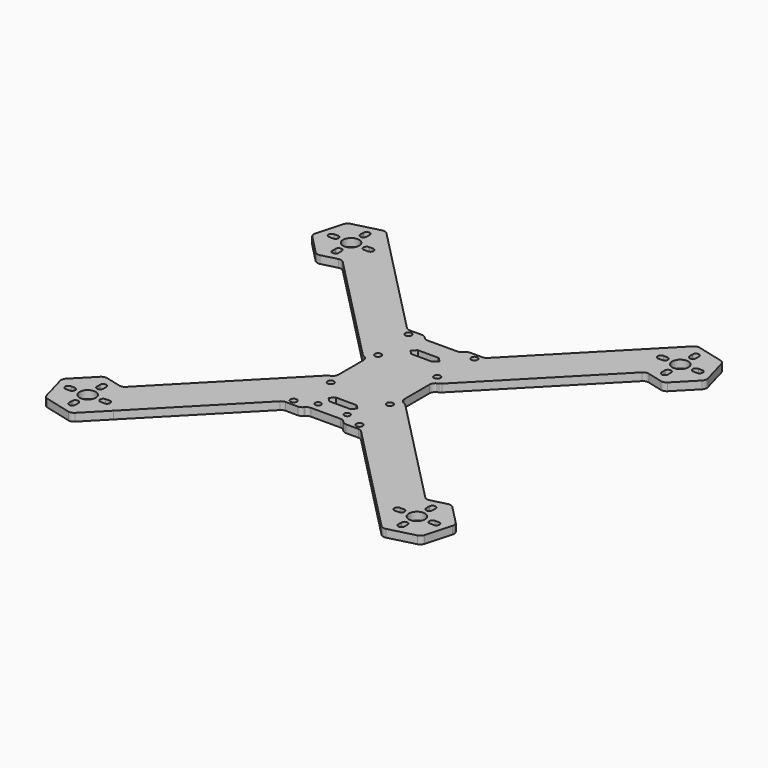
from build123d import *

# Parameters (mm, degrees)
F0_R     = 1.65
F0_R_2   = 4.15
F1_DEPTH = 4
F2_R     = 3
F5_R     = 1.5
F6_DEPTH = 43.5


# Not quite as in the source:
# - a feature names something its author has since deleted; it is built from what else it names


with BuildPart() as f1:
    # F0 (on Top) → F1 (new body)
    with BuildSketch(Plane.XY):
        Polygon((20, 40), (14, 40), (11.0626053065, 40), (9, 37.6), (0, 37.6), (0, 28.5310465842), (5.3786796564, 28.5310465842), (7.5, 26.4097262407), (5.3786796564, 24.2884058971), (0, 24.2884058971), (0, 0), (17, 0), (17, 10), (20, 11.3973480558), (78.334668641, 71.0380709735), (72.7416933404, 72.4705375943), (68.0738878405, 89.1502136048), align=None)
        with Locations((15.25, 15.25)):
            Circle(F0_R, mode=Mode.SUBTRACT)
        with Locations((17, 37)):
            Circle(F0_R, mode=Mode.SUBTRACT)
        Polygon((80.1850082425, 101.5324897529), (68.0738878405, 89.1502136048), (72.7416933404, 72.4705375943), (78.334668641, 71.0380709735), (89.5206192423, 68.1731377319), (101.6317396443, 80.55541388), (96.9639341444, 97.2350898905), align=None)
        with BuildLine():
            ThreePointArc((83.2528137424, 76.8528137424), (84.8528137424, 78.4528137424), (86.4528137424, 76.8528137424))
            Line((86.4528137424, 76.8528137424), (86.4528137424, 76.2028137424))
            Line((86.4528137424, 76.2028137424), (86.4528137424, 75.3528137424))
            Line((86.4528137424, 75.3528137424), (86.4528137424, 74.8528137424))
            ThreePointArc((86.4528137424, 74.8528137424), (84.8528137424, 73.2528137424), (83.2528137424, 74.8528137424))
            Line((83.2528137424, 74.8528137424), (83.2528137424, 76.2028137424))
            Line((83.2528137424, 76.2028137424), (83.2528137424, 76.8528137424))
        make_face(mode=Mode.SUBTRACT)
        with BuildLine():
            ThreePointArc((76.8528137424, 86.4528137424), (78.4528137424, 84.8528137424), (76.8528137424, 83.2528137424))
            Line((76.8528137424, 83.2528137424), (76.2028137424, 83.2528137424))
            Line((76.2028137424, 83.2528137424), (75.3528137424, 83.2528137424))
            Line((75.3528137424, 83.2528137424), (74.8528137424, 83.2528137424))
            ThreePointArc((74.8528137424, 83.2528137424), (73.2528137424, 84.8528137424), (74.8528137424, 86.4528137424))
            Line((74.8528137424, 86.4528137424), (76.2028137424, 86.4528137424))
            Line((76.2028137424, 86.4528137424), (76.8528137424, 86.4528137424))
        make_face(mode=Mode.SUBTRACT)
        with Locations((84.8528137424, 84.8528137424)):
            Circle(F0_R_2, mode=Mode.SUBTRACT)
        with BuildLine():
            Line((93.5028137424, 83.2528137424), (92.8528137424, 83.2528137424))
            ThreePointArc((92.8528137424, 83.2528137424), (91.2528137424, 84.8528137424), (92.8528137424, 86.4528137424))
            Line((92.8528137424, 86.4528137424), (93.5028137424, 86.4528137424))
            Line((93.5028137424, 86.4528137424), (94.8528137424, 86.4528137424))
            ThreePointArc((94.8528137424, 86.4528137424), (96.4528137424, 84.8528137424), (94.8528137424, 83.2528137424))
            Line((94.8528137424, 83.2528137424), (94.3528137424, 83.2528137424))
            Line((94.3528137424, 83.2528137424), (93.5028137424, 83.2528137424))
        make_face(mode=Mode.SUBTRACT)
        with BuildLine():
            ThreePointArc((86.4528137424, 92.8528137424), (84.8528137424, 91.2528137424), (83.2528137424, 92.8528137424))
            Line((83.2528137424, 92.8528137424), (83.2528137424, 93.5028137424))
            Line((83.2528137424, 93.5028137424), (83.2528137424, 94.3528137424))
            Line((83.2528137424, 94.3528137424), (83.2528137424, 94.8528137424))
            ThreePointArc((83.2528137424, 94.8528137424), (84.8528137424, 96.4528137424), (86.4528137424, 94.8528137424))
            Line((86.4528137424, 94.8528137424), (86.4528137424, 94.3528137424))
            Line((86.4528137424, 94.3528137424), (86.4528137424, 93.5028137424))
            Line((86.4528137424, 93.5028137424), (86.4528137424, 92.8528137424))
        make_face(mode=Mode.SUBTRACT)
    extrude(amount=F1_DEPTH)

    # F2
    f2_edges = [f1.edges().sort_by_distance(p)[0] for p in [
        (20, 11.397348, 2),
        (78.334669, 71.038071, 2),
        (17, 10, 2),
        (89.520619, 68.173138, 2),
        (101.63174, 80.555414, 2),
        (96.963934, 97.23509, 2),
        (80.185008, 101.53249, 2),
        (20, 40, 2),
        (11.062605, 40, 2),
        (9, 37.6, 2),
    ]]
    fillet(f2_edges, radius=F2_R)

    # F3: F1 across plane


with BuildPart() as f1_1:
    add(f1.part)
    add(f1.part.mirror(Plane.YZ))

    # F4: F1 across plane


with BuildPart() as f1_2:
    add(f1_1.part)
    add(f1_1.part.mirror(Plane.XZ))

    # F5 (on face) → F6 (cut, symmetric)
    with BuildSketch(Plane.XY.offset(4)):
        with Locations((-7.5, -33.0655232921)):
            Circle(F5_R)
        with Locations((7.5, -33.0655232921)):
            Circle(F5_R)
    extrude(amount=F6_DEPTH, both=True, mode=Mode.SUBTRACT)


solid = f1_2.part
